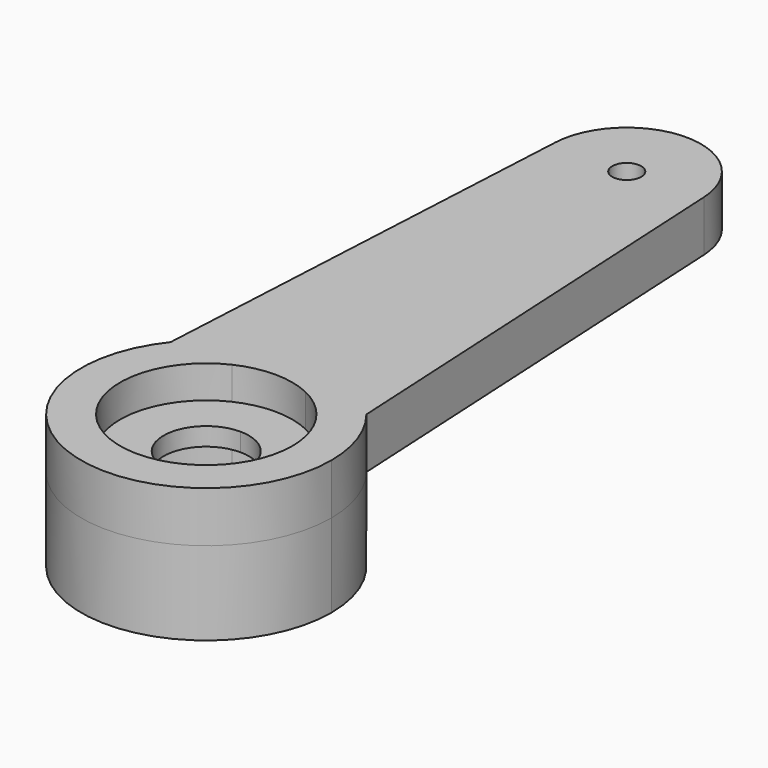
from build123d import *
from build123d import SkipClean  # not in build123d's __all__

# Parameters (mm, degrees)
F0_R     = 0.4
F1_DEPTH = 1.4
F2_DEPTH = 2.3
F3_DEPTH = 0.5


with BuildPart() as f1:
    # F0 (on Top) → F1 (new body)
    with BuildSketch(Plane.XY):
        with BuildLine():
            ThreePointArc((-2.7, 2.1476731595), (-1.1374313166, -3.2571076126), (3.45, 0))
            ThreePointArc((3.45, 0), (3.2571076126, 1.1374313166), (2.7, 2.1476731595))
            Line((2.7, 2.1476731595), (1.0139649895, 2.1476731595))
            ThreePointArc((1.0139649895, 2.1476731595), (2.0060897101, 1.2713099838), (2.375, 0))
            ThreePointArc((2.375, 0), (-1.2713099838, -2.0060897101), (-1.0139649895, 2.1476731595))
            Line((-1.0139649895, 2.1476731595), (-2.7, 2.1476731595))
        make_face()
        with BuildLine():
            Line((1.0139649895, 2.1476731595), (2.7, 2.1476731595))
            ThreePointArc((2.7, 2.1476731595), (0, 3.45), (-2.7, 2.1476731595))
            Line((-2.7, 2.1476731595), (-1.0139649895, 2.1476731595))
            ThreePointArc((-1.0139649895, 2.1476731595), (0, 2.375), (1.0139649895, 2.1476731595))
        make_face()
        with BuildLine():
            ThreePointArc((-2.7, 2.1476731595), (0, 3.45), (2.7, 2.1476731595))
            Line((2.7, 2.1476731595), (2.0471920173, 14.6072606371))
            ThreePointArc((2.0471920173, 14.6072606371), (2.0492978841, 14.553648693), (2.05, 14.5))
            ThreePointArc((2.05, 14.5), (-0.053648693, 12.4507021159), (-2.0471920173, 14.6072606371))
            Line((-2.0471920173, 14.6072606371), (-2.7, 2.1476731595))
        make_face()
        with BuildLine():
            ThreePointArc((2.05, 14.5), (2.0492978841, 14.553648693), (2.0471920173, 14.6072606371))
            ThreePointArc((2.0471920173, 14.6072606371), (0, 16.55), (-2.0471920173, 14.6072606371))
            ThreePointArc((-2.0471920173, 14.6072606371), (-0.053648693, 12.4507021159), (2.05, 14.5))
        make_face()
        with Locations((0, 14.5)):
            Circle(F0_R, mode=Mode.SUBTRACT)
    extrude(amount=F1_DEPTH)

    # F0 (on Top) → F2 (join)
    with BuildSketch(Plane.XY):
        with BuildLine():
            Line((1.0139649895, 2.1476731595), (2.7, 2.1476731595))
            ThreePointArc((2.7, 2.1476731595), (0, 3.45), (-2.7, 2.1476731595))
            Line((-2.7, 2.1476731595), (-1.0139649895, 2.1476731595))
            ThreePointArc((-1.0139649895, 2.1476731595), (0, 2.375), (1.0139649895, 2.1476731595))
        make_face()
        with BuildLine():
            ThreePointArc((-2.7, 2.1476731595), (-1.1374313166, -3.2571076126), (3.45, 0))
            ThreePointArc((3.45, 0), (3.2571076126, 1.1374313166), (2.7, 2.1476731595))
            Line((2.7, 2.1476731595), (1.0139649895, 2.1476731595))
            ThreePointArc((1.0139649895, 2.1476731595), (2.0060897101, 1.2713099838), (2.375, 0))
            ThreePointArc((2.375, 0), (-1.2713099838, -2.0060897101), (-1.0139649895, 2.1476731595))
            Line((-1.0139649895, 2.1476731595), (-2.7, 2.1476731595))
        make_face()
    with SkipClean():  # cleaning this boolean's faces spoils the solid; the shape is the same uncleaned
        extrude(amount=-F2_DEPTH)

    # F0 (on Top) → F3 (join)
    with BuildSketch(Plane.XY):
        with BuildLine():
            Line((0, 2.1476731595), (1.0139649895, 2.1476731595))
            ThreePointArc((1.0139649895, 2.1476731595), (0, 2.375), (-1.0139649895, 2.1476731595))
            Line((-1.0139649895, 2.1476731595), (0, 2.1476731595))
        make_face()
        with BuildLine():
            ThreePointArc((2.375, 0), (2.0060897101, 1.2713099838), (1.0139649895, 2.1476731595))
            Line((1.0139649895, 2.1476731595), (0, 2.1476731595))
            Line((0, 2.1476731595), (-1.0139649895, 2.1476731595))
            ThreePointArc((-1.0139649895, 2.1476731595), (-1.2713099838, -2.0060897101), (2.375, 0))
        make_face()
        with BuildLine():
            ThreePointArc((1.175, 0), (-0.8308504679, -0.8308504679), (0, 1.175))
            ThreePointArc((0, 1.175), (0.8308504679, 0.8308504679), (1.175, 0))
        make_face(mode=Mode.SUBTRACT)
    extrude(amount=F3_DEPTH)


solid = f1.part
